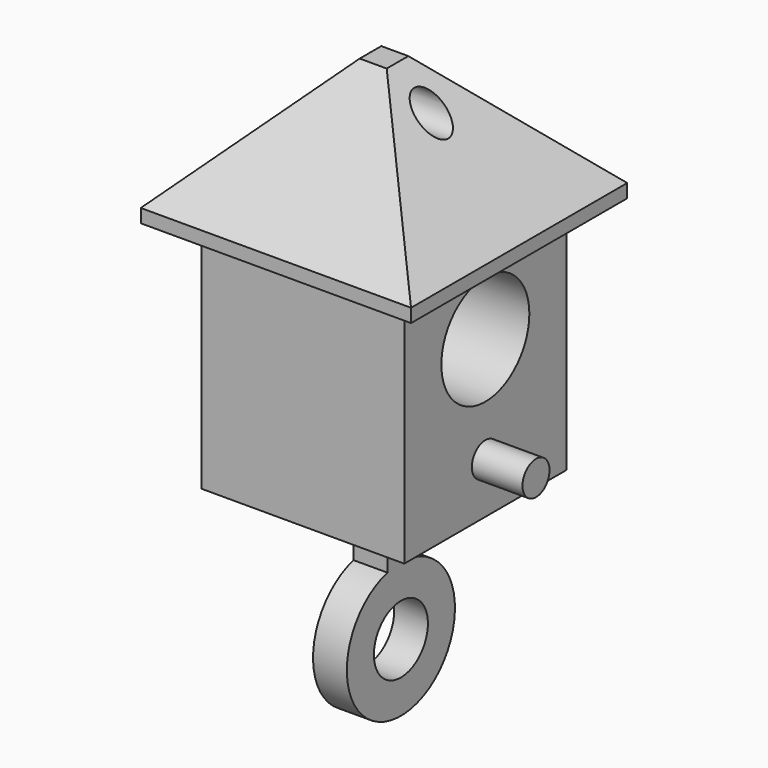
from build123d import *

# Parameters (mm, degrees)
F0_W      = 30
F0_H      = 30
F1_DEPTH  = 35
F2_W      = 40
F2_H      = 40
F3_DEPTH  = 20
F4_SIZE   = 18
F5_R      = 8.1403588374
F6_DEPTH  = 20
F7_R      = 2.5
F8_DEPTH  = 7.5
F9_R      = 2.5
F10_DEPTH = 79.502
F11_W     = 5
F11_H     = 5
F12_DEPTH = 15
F13_R     = 10
F13_R_2   = 5
F14_DEPTH = 2.5


# Not quite as in the source:
# - a feature names something its author has since deleted; it is built from what else it names


with BuildPart() as f1:
    # F0 (on Top) → F1 (new body)
    with BuildSketch(Plane.XY):
        Rectangle(F0_W, F0_H)
    extrude(amount=F1_DEPTH)

    # F2 (on face) → F3 (join)
    with BuildSketch(Plane.XY.offset(35)):
        Rectangle(F2_W, F2_H)
    extrude(amount=F3_DEPTH)

    # F4
    f4_edges = [f1.edges().sort_by_distance(p)[0] for p in [
        (20, 0, 55),
        (0, 20, 55),
        (-20, 0, 55),
        (0, -20, 55),
    ]]
    chamfer(f4_edges, length=F4_SIZE)

    # F5 (on face) → F6 (cut)
    with BuildSketch(Plane.YZ.offset(15)):
        with Locations((0, 23.1403588374)):
            Circle(F5_R)
    extrude(amount=-F6_DEPTH, mode=Mode.SUBTRACT)

    # F7 (on face) → F8 (join)
    with BuildSketch(Plane.YZ.offset(15)):
        with Locations((0, 7.5)):
            Circle(F7_R)
    extrude(amount=F8_DEPTH)

    # F9 (on face) → F10 (cut)
    with BuildSketch(Plane.YZ.offset(20)):
        with Locations((0, 50)):
            Circle(F9_R)
    extrude(amount=-F10_DEPTH, mode=Mode.SUBTRACT)

    # F11 (on face) → F12 (join)
    with BuildSketch(Plane(origin=(0, 0, 0), x_dir=(1, 0, 0), z_dir=(0, 0, -1))):
        Rectangle(F11_W, F11_H)
    extrude(amount=F12_DEPTH)

    # F13 (on Right) → F14 (join, symmetric)
    with BuildSketch(Plane.YZ):
        with Locations((0, -20)):
            Circle(F13_R)
        with Locations((0, -20)):
            Circle(F13_R_2, mode=Mode.SUBTRACT)
    extrude(amount=F14_DEPTH, both=True)


solid = f1.part
